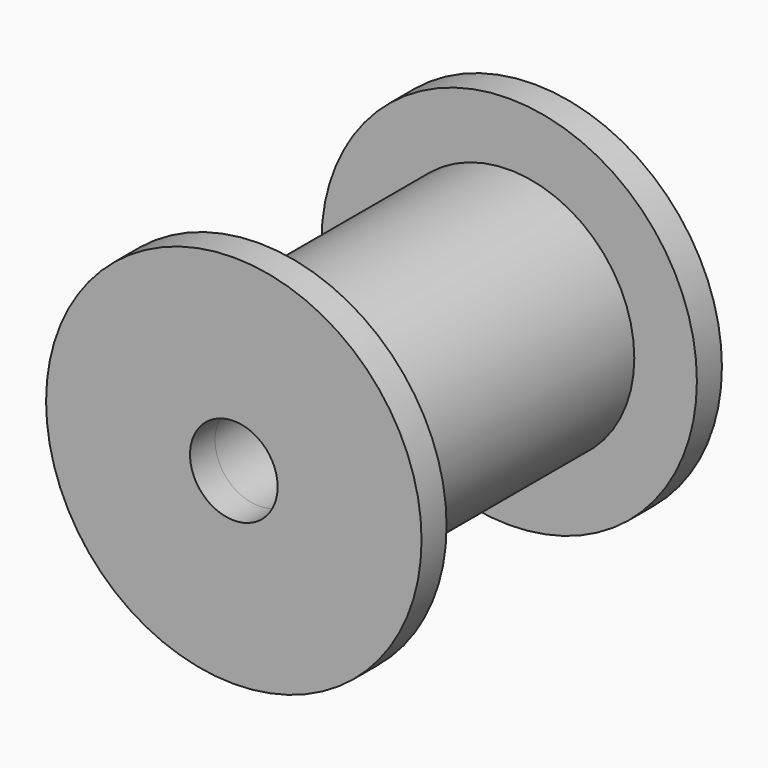
from build123d import *

# Parameters (mm, degrees)
F0_R     = 20
F0_R_2   = 7
F1_DEPTH = 25
F2_R     = 30
F2_R_2   = 7
F3_DEPTH = 5


with BuildPart() as f1:
    # F0 (on Front) → F1 (new body, symmetric)
    with BuildSketch(Plane.XZ):
        Circle(F0_R)
        Circle(F0_R_2, mode=Mode.SUBTRACT)
    extrude(amount=F1_DEPTH, both=True)

    # F2 (on face) → F3 (join)
    with BuildSketch(Plane.XZ.offset(25)):
        Circle(F2_R)
        Circle(F2_R_2, mode=Mode.SUBTRACT)
    extrude(amount=F3_DEPTH)

    # F4: F1 across plane


with BuildPart() as f1_1:
    add(f1.part)
    add(f1.part.mirror(Plane.XZ))


solid = f1_1.part
